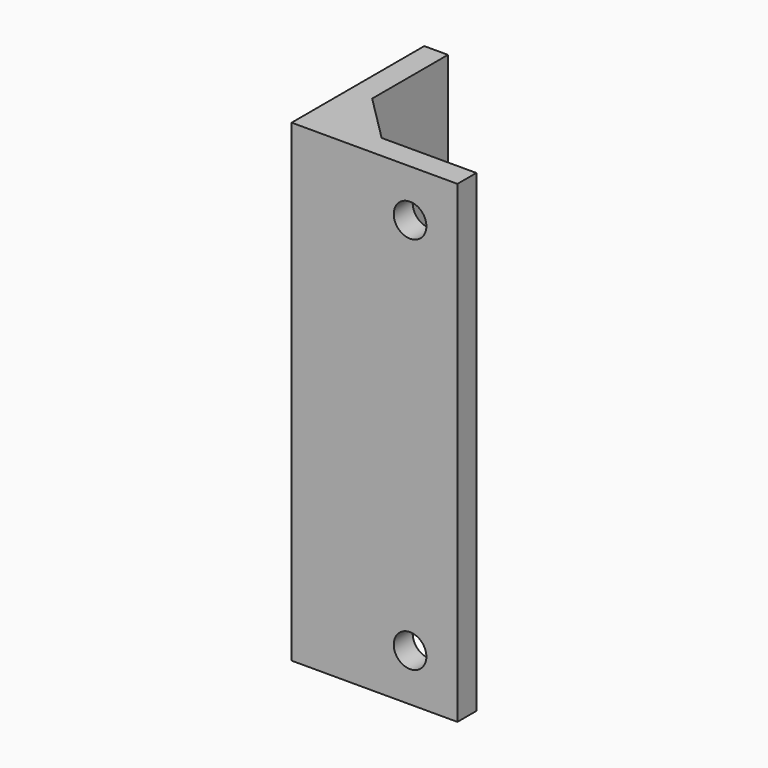
from build123d import *

# Parameters (mm, degrees)
F1_DEPTH    = 50.8
F2_R        = 1.75
F3_DEPTH    = 25.4
F5_T4_DEPTH = 50.8
F5_S5_R     = 1.75
F5_T6_DEPTH = 27
F5_S7_R     = 1.75
F5_T8_DEPTH = 27
F2_R_2      = 3
F6_DEPTH    = 7.511
F7_DEPTH    = 2.54
F4_R        = 1.75
F8_DEPTH    = 2.54


# Not quite as in the source:
# - a fillet or chamfer that OpenCascade refuses, or shapes differently, is made with other operations: its cross-section is extruded or revolved along the edge and cut away or added


with BuildPart() as f1:
    # F0 (on Top) → F1 (new body)
    with BuildSketch(Plane.XY):
        Polygon((0, 17.78), (0, 0), (17.78, 0), (17.78, 2.54), (2.54, 2.54), (2.54, 17.78), align=None)
    extrude(amount=F1_DEPTH)

    # F2 (on face) → F3 (cut)
    with BuildSketch(Plane(origin=(0, 0, 0), x_dir=(0, -1, 0), z_dir=(-1, 0, 0))):
        with Locations((-5.65, 9.9)):
            Circle(F2_R)
        with Locations((-5.65, 40.9)):
            Circle(F2_R)
    extrude(amount=-F3_DEPTH, mode=Mode.SUBTRACT)

    # F5: chamfer of 5.08 on 1 edges, made by hand


with BuildPart() as f5_tool2:
    # F5_s3 → F5_t4 (new body)
    with BuildSketch(Plane.XY):
        Polygon((2.54, 7.62), (7.62, 2.54), (2.54, 2.54), align=None)
    extrude(amount=F5_T4_DEPTH)

    # F5_s5 → F5_t6 (cut, symmetric)
    with BuildSketch(Plane.YZ.offset(5.1)):
        with Locations((5.65, 40.9)):
            Circle(F5_S5_R)
    extrude(amount=F5_T6_DEPTH, both=True, mode=Mode.SUBTRACT)

    # F5_s7 → F5_t8 (cut, symmetric)
    with BuildSketch(Plane.YZ.offset(5.1)):
        with Locations((5.65, 9.9)):
            Circle(F5_S7_R)
    extrude(amount=F5_T8_DEPTH, both=True, mode=Mode.SUBTRACT)


with BuildPart() as f1_1:
    add(f1.part)

    # F5_t1: union F5_tool2
    add(f5_tool2.part)

    # F2 (on face) → F6 (cut, through all)
    with BuildSketch(Plane(origin=(0, 0, 0), x_dir=(0, -1, 0), z_dir=(-1, 0, 0))):
        with Locations((-5.65, 40.9)):
            Circle(F2_R_2)
        with Locations((-5.65, 40.9)):
            Circle(F2_R, mode=Mode.SUBTRACT)
        with Locations((-5.65, 9.9)):
            Circle(F2_R_2)
        with Locations((-5.65, 9.9)):
            Circle(F2_R, mode=Mode.SUBTRACT)
    extrude(amount=-F6_DEPTH, mode=Mode.SUBTRACT)

    # F2 (on face) → F7 (join)
    with BuildSketch(Plane(origin=(0, 0, 0), x_dir=(0, -1, 0), z_dir=(-1, 0, 0))):
        with Locations((-5.65, 40.9)):
            Circle(F2_R_2)
        with Locations((-5.65, 40.9)):
            Circle(F2_R, mode=Mode.SUBTRACT)
        with Locations((-5.65, 9.9)):
            Circle(F2_R_2)
        with Locations((-5.65, 9.9)):
            Circle(F2_R, mode=Mode.SUBTRACT)
    extrude(amount=-F7_DEPTH)

    # F4 (on face) → F8 (cut, through all)
    with BuildSketch(Plane.XZ):
        with Locations((12.7, 45.72)):
            Circle(F4_R)
        with Locations((12.7, 5.08)):
            Circle(F4_R)
    extrude(amount=-F8_DEPTH, mode=Mode.SUBTRACT)


solid = f1_1.part
